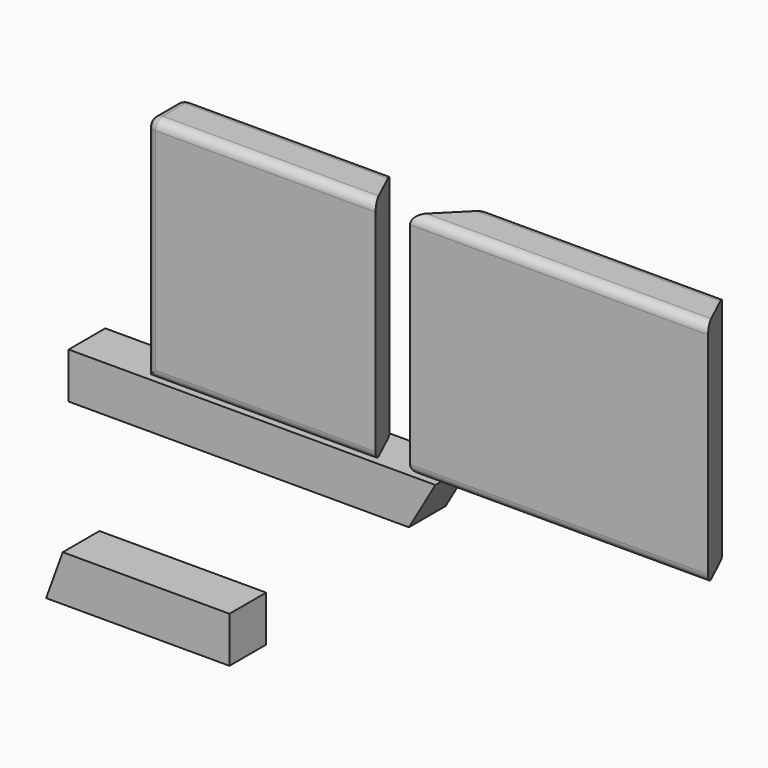
from build123d import *

# Parameters (mm, degrees)
F0_W      = 127
F0_H      = 127
F1_DEPTH  = 25.4
F2_SIZE2  = 11.844205
F2_SIZE   = 25.39999
F3_W      = 165.1
F3_H      = 127
F4_DEPTH  = 25.4
F5_SIZE2  = 11.844205
F5_SIZE   = 25.39999
F6_SIZE2  = 25.39999
F6_SIZE   = 25.39999
F7_W      = 203.2
F7_H      = 25.4
F8_DEPTH  = 25.4
F9_SIZE2  = 14.664687
F9_SIZE   = 25.39999
F10_R     = 5.08
F10_2_R   = 5.08
F11_W     = 101.6
F11_H     = 25.4
F12_DEPTH = 25.4
F13_SIZE2 = 9.244834
F13_SIZE  = 25.39999


# Not quite as in the source:
# - a fillet or chamfer is up to 0.001 mm smaller than in the source, because OpenCascade refuses the exact size


with BuildPart() as f1:
    # F0 (on Front) → F1 (new body)
    with BuildSketch(Plane.XZ):
        with Locations((63.5, 63.5)):
            Rectangle(F0_W, F0_H)
    extrude(amount=F1_DEPTH)

    # F2 (size 25.4 and 11.8442145171 in the source; OpenCascade refuses exactly that, so slightly less here)
    f2_edges = [f1.edges().sort_by_distance(p)[0] for p in [
        (127, 0, 63.5),
    ]]
    f2_side = f1.faces().sort_by_distance((127, -12.7, 63.5))[0]
    chamfer(f2_edges, length=F2_SIZE, length2=F2_SIZE2, reference=f2_side)

    # F10
    f10_edges = [f1.edges().sort_by_distance(p)[0] for p in [
        (63.5, -25.4, 127),
        (57.577898, 0, 127),
        (0, -25.4, 63.5),
        (0, -12.7, 127),
        (63.5, -25.4, 0),
        (115.155795, 0, 63.5),
        (57.577897, 0, 0),
        (0, 0, 63.5),
    ]]
    fillet(f10_edges, radius=F10_R)


with BuildPart() as f4:
    # F3 (on Front) → F4 (new body)
    with BuildSketch(Plane.XZ):
        with Locations((228.6448437452, 63.5)):
            Rectangle(F3_W, F3_H)
    extrude(amount=F4_DEPTH)

    # F5 (size 25.4 and 11.8442145171 in the source; OpenCascade refuses exactly that, so slightly less here)
    f5_edges = [f4.edges().sort_by_distance(p)[0] for p in [
        (311.194844, 0, 63.5),
    ]]
    f5_side = f4.faces().sort_by_distance((311.194844, -12.7, 63.5))[0]
    chamfer(f5_edges, length=F5_SIZE, length2=F5_SIZE2, reference=f5_side)

    # F6 (size 25.4 and 25.4 in the source; OpenCascade refuses exactly that, so slightly less here)
    f6_edges = [f4.edges().sort_by_distance(p)[0] for p in [
        (146.094844, 0, 63.5),
    ]]
    chamfer(f6_edges, length=F6_SIZE, length2=F6_SIZE2)

    # F10#2
    f10_2_edges = [f4.edges().sort_by_distance(p)[0] for p in [
        (235.422736, 0, 0),
        (299.350639, 0, 63.5),
        (235.422736, 0, 127),
        (228.644844, -25.4, 127),
        (228.644844, -25.4, 0),
    ]]
    fillet(f10_2_edges, radius=F10_2_R)


with BuildPart() as f8:
    # F7 (on face) → F8 (new body)
    with BuildSketch(Plane(origin=(0, 0, 0), x_dir=(-1, 0, 0), z_dir=(0, 1, 0))):
        with Locations((-38.2195329294, -30.0378452635)):
            Rectangle(F7_W, F7_H)
    extrude(amount=F8_DEPTH)

    # F9 (size 25.4 and 14.6646968374 in the source; OpenCascade refuses exactly that, so slightly less here)
    f9_edges = [f8.edges().sort_by_distance(p)[0] for p in [
        (139.819533, 12.7, -42.737845),
    ]]
    f9_side = f8.faces().sort_by_distance((139.819533, 12.7, -30.037845))[0]
    chamfer(f9_edges, length=F9_SIZE, length2=F9_SIZE2, reference=f9_side)


with BuildPart() as f12:
    # F11 (on Front) → F12 (new body)
    with BuildSketch(Plane.XZ):
        with Locations((-4.744283855, -113.0070951225)):
            Rectangle(F11_W, F11_H)
    extrude(amount=F12_DEPTH)

    # F13 (size 25.4 and 9.2448439504 in the source; OpenCascade refuses exactly that, so slightly less here)
    f13_edges = [f12.edges().sort_by_distance(p)[0] for p in [
        (-55.544284, -12.7, -100.307095),
    ]]
    f13_side = f12.faces().sort_by_distance((-55.544284, -12.7, -113.007095))[0]
    chamfer(f13_edges, length=F13_SIZE, length2=F13_SIZE2, reference=f13_side)


solid = Compound([f1.part, f4.part, f8.part, f12.part])
